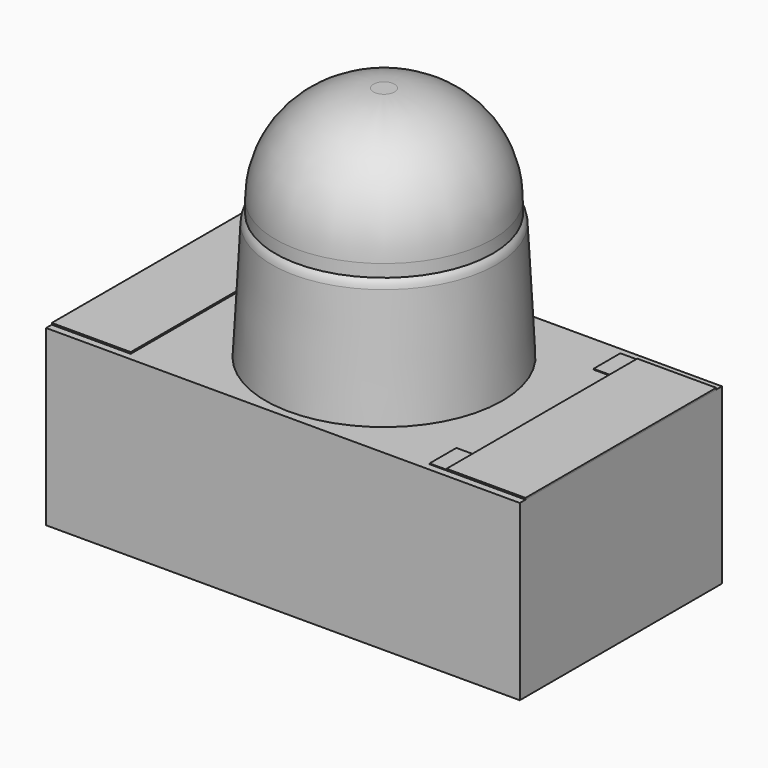
from build123d import *

# Parameters (mm, degrees)
F0_W      = 0.5
F0_H      = 1.5099706361
F0_R      = 0.7493333287
F0_W_2    = 0.1072544944
F0_H_2    = 0.2120600548
F1_DEPTH  = 1.1
F2_DEPTH  = 0.8
F2_TAPER  = 3
F4_DEPTH  = 0.01
F5_DEPTH  = 0.005
F3_R      = 0.6874071052
F6_DEPTH  = 0.7
F7_R      = 0.6204528855
F9_W      = 0.9084290941
F9_H      = 1.1024641572
F10_DEPTH = 0.01


# Not quite as in the source:
# - a fillet or chamfer that OpenCascade refuses, or shapes differently, is made with other operations: its cross-section is extruded or revolved along the edge and cut away or added


with BuildPart() as f1:
    # F0 (on Top) → F1 (new body)
    with BuildSketch(Plane.XY):
        with Locations((-1.25, 0)):
            Rectangle(F0_W, F0_H)
        Polygon((-1.5, -0.8), (1.5, -0.8), (1.5, -0.7549853181), (1, -0.7549853181), (0.8927455056, -0.7549853181), (0.8927455056, -0.5429252633), (1, -0.5429252633), (1, 0.5429252633), (0.8927455056, 0.5429252633), (0.8927455056, 0.7549853181), (1, 0.7549853181), (1.5, 0.7549853181), (1.5, 0.8), (-1.5, 0.8), (-1.5, 0.7549853181), (-1, 0.7549853181), (-1, -0.7549853181), (-1.5, -0.7549853181), align=None)
        Circle(F0_R, mode=Mode.SUBTRACT)
        Circle(F0_R)
        with Locations((0.9463727528, 0.6489552907)):
            Rectangle(F0_W_2, F0_H_2)
        Polygon((1, -0.7549853181), (1.5, -0.7549853181), (1.5, 0.7549853181), (1, 0.7549853181), (1, 0.5429252633), (1, -0.5429252633), align=None)
        with Locations((0.9463727528, -0.6489552907)):
            Rectangle(F0_W_2, F0_H_2)
    extrude(amount=-F1_DEPTH)


with BuildPart() as f2:
    # F0 (on Top) → F2 (new body)
    with BuildSketch(Plane.XY):
        Circle(F0_R)
    extrude(amount=F2_DEPTH, taper=F2_TAPER)

    # F3 (on face) → F6 (join)
    with BuildSketch(Plane.XY.offset(0.8)):
        Circle(F3_R)
    extrude(amount=F6_DEPTH)

    # F7
    f7_edges = [f2.edges().sort_by_distance(p)[0] for p in [
        (-0.687407, 0, 1.5),
    ]]
    fillet(f7_edges, radius=F7_R)

    # F8: fillet of radius 0.0871635846 on 1 edges, made by hand

    # F8_s1 → F8_t2 (revolve, cut)
    with BuildSketch(Plane.XZ):
        with BuildLine():
            ThreePointArc((0.6874071052, 0.8), (0.703576177, 0.7747914026), (0.7102582005, 0.7455978618))
            Line((0.7102582005, 0.7455978618), (0.7074071052, 0.8))
            Line((0.7074071052, 0.8), (0.6874071052, 0.8))
        make_face()
    revolve(axis=Axis((0, 0, 0.8), (0, 0, -1)), mode=Mode.SUBTRACT)


with BuildPart() as f4:
    # F0 (on Top) → F4 (new body)
    with BuildSketch(Plane.XY):
        with Locations((-1.25, 0)):
            Rectangle(F0_W, F0_H)
    extrude(amount=F4_DEPTH)


with BuildPart() as f4b:
    # F0 (on Top) → F4, piece 2 (new body)
    with BuildSketch(Plane.XY):
        Polygon((1, -0.7549853181), (1.5, -0.7549853181), (1.5, 0.7549853181), (1, 0.7549853181), (1, 0.5429252633), (1, -0.5429252633), align=None)
    extrude(amount=F4_DEPTH)


with BuildPart() as f5:
    # F0 (on Top) → F5 (new body)
    with BuildSketch(Plane.XY):
        with Locations((0.9463727528, -0.6489552907)):
            Rectangle(F0_W_2, F0_H_2)
    extrude(amount=F5_DEPTH)


with BuildPart() as f5b:
    # F0 (on Top) → F5, piece 2 (new body)
    with BuildSketch(Plane.XY):
        with Locations((0.9463727528, 0.6489552907)):
            Rectangle(F0_W_2, F0_H_2)
    extrude(amount=F5_DEPTH)


with BuildPart() as f10:
    # F9 (on face) → F10 (new body)
    with BuildSketch(Plane(origin=(0, 0, -1.1), x_dir=(1, 0, 0), z_dir=(0, 0, -1))):
        with Locations((-0.8086880553, 0)):
            Rectangle(F9_W, F9_H)
    extrude(amount=F10_DEPTH)


solid = Compound([f1.part, f2.part, f4.part, f4b.part, f5.part, f5b.part, f10.part])
